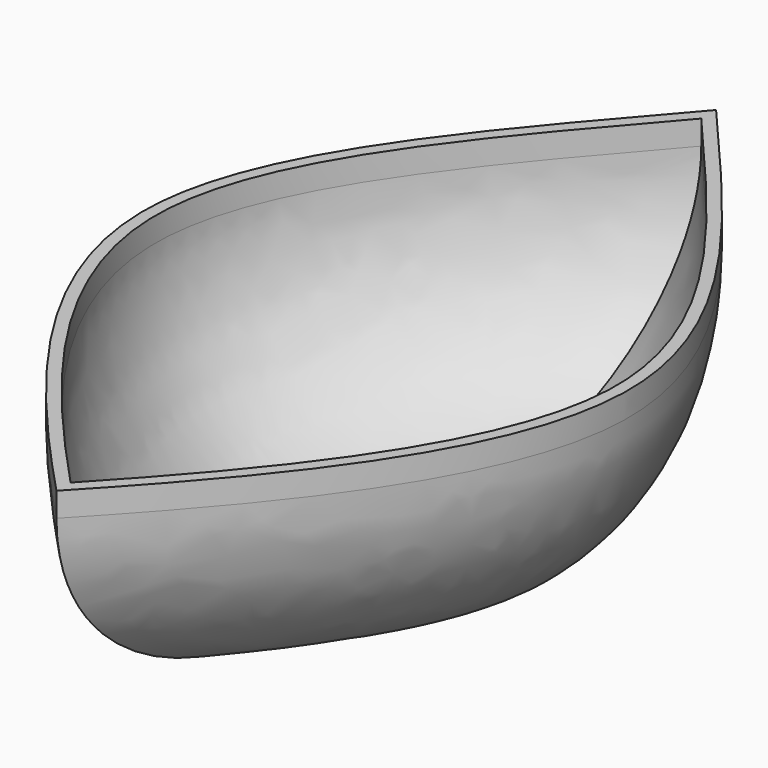
from build123d import *

# Parameters (mm, degrees)
F1_DEPTH = 25.4
F2_R     = 22.86
F3_T     = 1.27


# Not quite as in the source:
# - a shell that OpenCascade refuses in one call is made with other operations: the cavity is built on its own and cut out


with BuildPart() as f1:
    # F0 (on Top) → F1 (new body)
    with BuildSketch(Plane.XY):
        with BuildLine():
            add(Edge.make_bspline(
                [(0, 43.18), (12.6277618203, 28.5479942033), (38.1078160952, 0.5540033901), (12.7566059893, -29.6560009835), (0, -43.18)],
                knots=[0, 0, 0, 0, 0.5, 1, 1, 1, 1], degree=3))
            add(Edge.make_bspline(
                [(0, 43.18), (-12.6384950786, 28.547848961), (-38.0970572555, 0.5541481006), (-12.7673904104, -29.6561451622), (0, -43.18)],
                knots=[0, 0, 0, 0, 0.5, 1, 1, 1, 1], degree=3))
        make_face()
    extrude(amount=F1_DEPTH)

    # F2
    f2_edges = [f1.edges().sort_by_distance(p)[0] for p in [
        (25.400061, -0.050271, 0),
        (-25.400061, -0.050358, 0),
    ]]
    fillet(f2_edges, radius=F2_R)

    # F3: shell of thickness 1.27, made by hand


with BuildPart() as f3_core1:
    # F3_t2: copy of F1
    add(f1.part)

    # the walls: a layer under each face that stays
    f3_faces = [f3_core1.faces().sort_by_distance(p)[0] for p in [
        (25.4, 0, 24.1299999999),
        (-25.4, 0, 24.1299999999),
        (18.704477423, -0.0148216465, 6.6955389821),
        (-18.704477436, -0.0148275323, 6.6955389821),
        (-1.3114e-06, -0.2233707907, 0),
    ]]
    thicken(f3_faces, amount=-F3_T, mode=Mode.SUBTRACT)


with BuildPart() as f1_1:
    add(f1.part)

    # what is left inside the walls is the cavity
    f3_cavity = [f3_core1.part.solids().sort_by_distance(p)[0] for p in [
        (-2e-06, -13.805023, 25.3873),
    ]]
    add(f3_cavity, mode=Mode.SUBTRACT)


solid = f1_1.part
